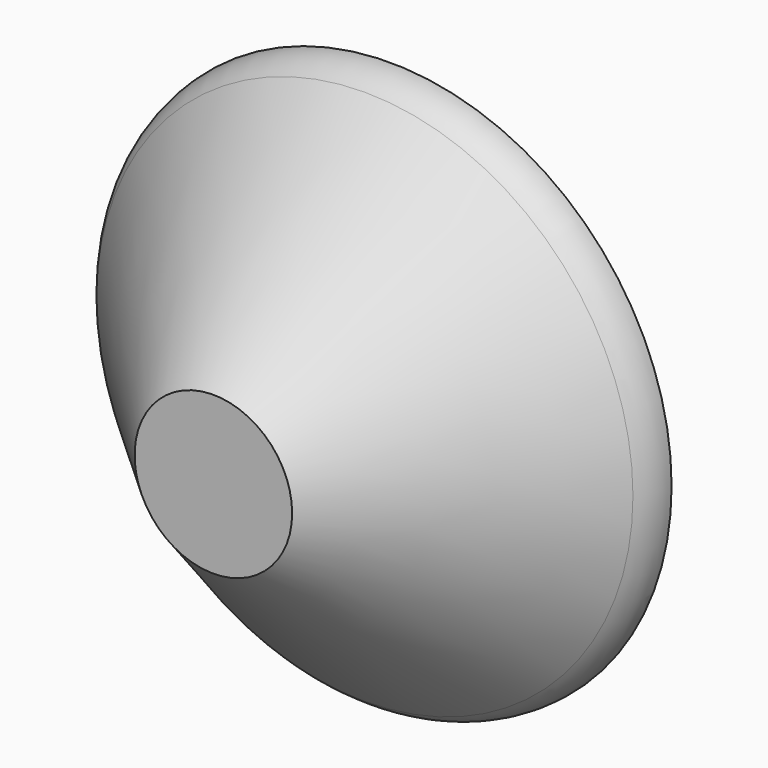
from build123d import *

# Parameters (mm, degrees)
F0_R     = 31.75
F1_DEPTH = 25.4
F2_SIZE  = 22.86
F5_T     = -1.27


# Not quite as in the source:
# - a fillet or chamfer that OpenCascade refuses, or shapes differently, is made with other operations: its cross-section is extruded or revolved along the edge and cut away or added
# - a feature of the source that left no trace in its solid (it failed there, or was rolled back) is left out
# - a shell that OpenCascade refuses in one call is made with other operations: the cavity is built on its own and cut out


with BuildPart() as f1:
    # F0 (on Front) → F1 (new body)
    with BuildSketch(Plane.XZ):
        Circle(F0_R)
    extrude(amount=F1_DEPTH)

    # F2
    f2_edges = [f1.edges().sort_by_distance(p)[0] for p in [
        (-31.75, -25.4, 0),
    ]]
    chamfer(f2_edges, length=F2_SIZE)

    # F4: fillet of radius 5.08 on 2 edges, made by hand

    # F4_s1 → F4_t2 (revolve, cut)
    with BuildSketch(Plane.XY):
        with BuildLine():
            ThreePointArc((31.75, -0.4357951031), (31.3633080252, -2.3798269396), (30.2621024484, -4.0278975516))
            Line((30.2621024484, -4.0278975516), (31.75, -2.54))
            Line((31.75, -2.54), (31.75, -0.4357951031))
        make_face()
    revolve(axis=Axis((0, -2.54, 0), (0, -1, 0)), mode=Mode.SUBTRACT)

    # F4_s3 → F4_t4 (revolve, cut)
    with BuildSketch(Plane.XY):
        with BuildLine():
            ThreePointArc((31.75, -0.4357951031), (30.7435201994, -0.1101428151), (29.691417751, 0))
            Line((29.691417751, 0), (31.75, 0))
            Line((31.75, 0), (31.75, -0.4357951031))
        make_face()
    revolve(axis=Axis((0, 0, 0), (0, -1, 0)), mode=Mode.SUBTRACT)

    # F5: a shell. OpenCascade refuses it in one call, so the cavity is built on its own and cut out:
    # the body offset inwards by the wall thickness, plus a prism from it out through each open face.
    f5_core = offset(f1.part, amount=F5_T, mode=Mode.PRIVATE)
    f5_exits = [f5_core.faces().sort_by_distance(p)[0] for p in [
        (0, -1.27, 0),
    ]]
    add(f5_core, mode=Mode.SUBTRACT)
    extrude(f5_exits, amount=-F5_T, mode=Mode.SUBTRACT)


solid = f1.part
